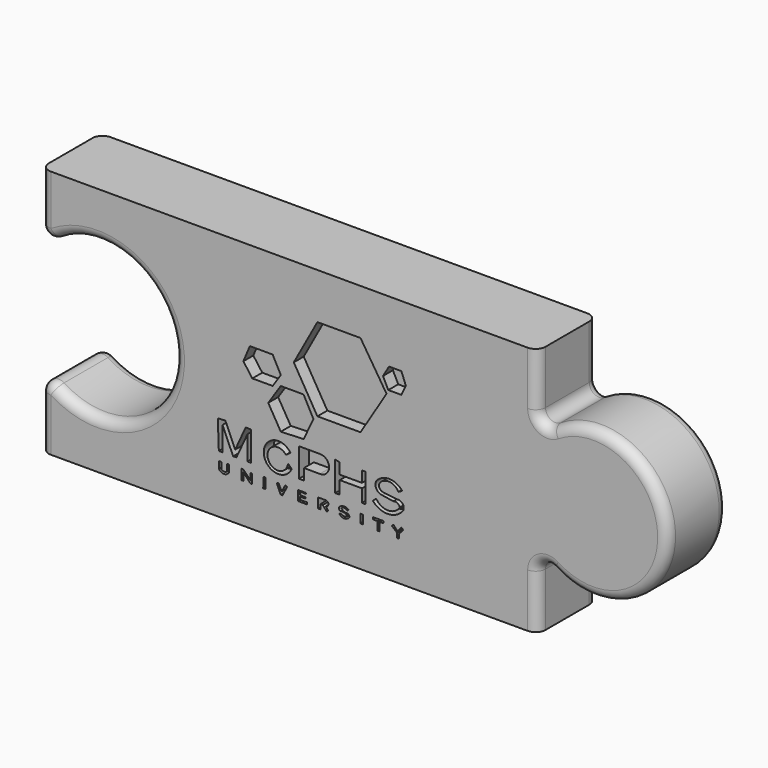
from build123d import *

# Parameters (mm, degrees)
F0_W     = 1.2396853417
F0_H     = 4.4274516404
F1_DEPTH = 38.1
F2_W     = 119.5903643966
F2_H     = 100.5869656801
F3_DEPTH = 31.75
F4_R     = 5.08
F5_F1_R  = 5.08
F5_F2_R  = 5.08


with BuildPart() as f1:
    # F0 (on Front) → F1 (new body)
    with BuildSketch(Plane.XZ):
        with BuildLine():
            Line((-152.3589964796, -18.4749997108), (-152.3589964796, -56.1939997108))
            Line((-152.3589964796, -56.1939997108), (101.6410035204, -56.1939997108))
            Line((101.6410035204, -56.1939997108), (101.6410035204, -17.8399997108))
            ThreePointArc((101.6410035204, -17.8399997108), (168.1390668347, 7.5600002892), (101.6410035204, 32.9600002892))
            Line((101.6410035204, 32.9600002892), (101.6410035204, 71.3140002892))
            Line((101.6410035204, 71.3140002892), (-152.3589964796, 71.3140002892))
            Line((-152.3589964796, 71.3140002892), (-152.3589964796, 34.8650002892))
            ThreePointArc((-152.3589964796, 34.8650002892), (-84.0285406821, 8.1950002892), (-152.3589964796, -18.4749997108))
        make_face()
        with BuildLine():
            Line((-61.3174373154, -34.5783394995), (-61.3174373154, -31.0568188551))
            Line((-61.3174373154, -31.0568188551), (-59.9337452893, -31.0568188551))
            Line((-59.9337452893, -31.0568188551), (-59.9337452893, -34.5783394995))
            ThreePointArc((-59.9337452893, -34.5783394995), (-58.6214708035, -34.9750876834), (-57.3091963177, -34.5783394995))
            Line((-57.3091963177, -34.5783394995), (-57.3091963177, -30.9339215281))
            Line((-57.3091963177, -30.9339215281), (-56.2031091993, -30.9339215281))
            Line((-56.2031091993, -30.9339215281), (-56.2031091993, -34.5783394995))
            ThreePointArc((-56.2031091993, -34.5783394995), (-58.7602732574, -36.0604791286), (-61.3174373154, -34.5783394995))
        make_face(mode=Mode.SUBTRACT)
        Polygon((-48.8504106049, -35.9585632804), (-49.8641850297, -35.9585632804), (-49.8641850297, -30.6131218794), (-48.8504106049, -30.7326440933), (-45.1566809659, -34.6184236231), (-45.1566809659, -31.1815415743), (-44.4813379888, -31.1815415743), (-44.4813379888, -35.9585632804), (-45.1566809659, -35.9585632804), (-48.8504106049, -32.0727837506), align=None, mode=Mode.SUBTRACT)
        Polygon((-37.5808859114, -35.9585632804), (-38.6635968332, -35.9585632804), (-38.5687844698, -30.7326440933), (-37.5808859114, -30.7326440933), align=None, mode=Mode.SUBTRACT)
        Polygon((-29.7552277202, -35.9585632804), (-31.7678497975, -31.3914579573), (-30.8955507223, -30.9392227448), (-29.1933210332, -34.3822178983), (-27.3931425903, -30.9392227448), (-26.4644501601, -31.4247918549), (-28.8349436466, -35.9585632804), align=None, mode=Mode.SUBTRACT)
        Polygon((-20.9552533795, -35.9585632804), (-20.9552533795, -30.9392227448), (-16.7476162185, -30.9392227448), (-16.7476162185, -31.4247918549), (-19.9163230006, -31.3914579573), (-19.9163230006, -32.909591985), (-16.9652923812, -32.909591985), (-16.9652923812, -33.6100806716), (-19.9163230006, -33.6100806716), (-19.9163230006, -35.0115646842), (-16.2226064001, -35.0115646842), (-16.2226064001, -35.9585632804), align=None, mode=Mode.SUBTRACT)
        with BuildLine():
            Line((-9.4527713825, -35.9585632804), (-10.54931454, -35.9585632804))
            Line((-10.54931454, -35.9585632804), (-10.54931454, -30.9392227448))
            Line((-10.54931454, -30.9392227448), (-6.6861817484, -30.9392227448))
            ThreePointArc((-6.6861817484, -30.9392227448), (-5.350752785, -32.2746517082), (-6.6861817484, -33.6100806716))
            Line((-6.6861817484, -33.6100806716), (-5.4284043645, -35.3105601402))
            Line((-5.4284043645, -35.3105601402), (-6.1631419683, -35.9585632804))
            Line((-6.1631419683, -35.9585632804), (-8.2343903939, -33.6100806716))
            Line((-8.2343903939, -33.6100806716), (-9.4527713825, -33.6100806716))
            Line((-9.4527713825, -33.6100806716), (-9.4527713825, -35.9585632804))
        make_face(mode=Mode.SUBTRACT)
        with BuildLine():
            ThreePointArc((4.3687420095, -35.5939765694), (2.0619009939, -36.0086349443), (0.2136342357, -34.5673275414))
            Line((0.2136342357, -34.5673275414), (1.3034986462, -34.5673275414))
            ThreePointArc((1.3034986462, -34.5673275414), (2.8361203279, -35.1923128719), (4.3687420095, -34.5673275414))
            ThreePointArc((4.3687420095, -34.5673275414), (2.9887125934, -33.5661164344), (1.3034986462, -33.3073524061))
            ThreePointArc((1.3034986462, -33.3073524061), (0.1017785642, -32.763786194), (0.4861005711, -31.502084178))
            ThreePointArc((0.4861005711, -31.502084178), (2.7680040932, -30.6538359895), (5.0499076153, -31.502084178))
            Line((5.0499076153, -31.502084178), (4.232510006, -32.0470159176))
            ThreePointArc((4.232510006, -32.0470159176), (2.7680043261, -31.2866876701), (1.3034986462, -32.0470159176))
            ThreePointArc((1.3034986462, -32.0470159176), (2.6880494547, -33.0373048641), (4.3687420095, -33.3073524061))
            ThreePointArc((4.3687420095, -33.3073524061), (5.3689469814, -34.4506644878), (4.3687420095, -35.5939765694))
        make_face(mode=Mode.SUBTRACT)
        Polygon((-59.4914490227, -26.5673523071), (-61.374177212, -26.5673523071), (-61.8983199651, -11.9427057781), (-58.0314019255, -11.8041166462), (-53.0015187031, -23.2180858651), (-47.6415390077, -11.5055379691), (-44.8480220382, -11.5055379691), (-44.8480220382, -26.5673523071), (-46.7307465021, -26.5673523071), (-46.7307465021, -14.225031552), (-52.3789273445, -26.5673523071), (-54.0524618571, -26.5673523071), (-59.4914490227, -14.225031552), align=None, mode=Mode.SUBTRACT)
        with BuildLine():
            ThreePointArc((-24.1380287205, -22.5927059772), (-38.3714144128, -20.264640143), (-24.7656023, -15.4801824364))
            Line((-24.7656023, -15.4801824364), (-27.0667122547, -17.1537188115))
            ThreePointArc((-27.0667122547, -17.1537188115), (-36.2738173156, -21.7936388182), (-26.0207531844, -20.7099796506))
            Line((-26.0207531844, -20.7099796506), (-24.1380287205, -22.5927059772))
        make_face(mode=Mode.SUBTRACT)
        with BuildLine():
            Line((-17.8622696419, -20.0775365629), (-17.8622696419, -25.7305850509))
            Line((-17.8622696419, -25.7305850509), (-20.3725714107, -25.7305850509))
            Line((-20.3725714107, -25.7305850509), (-20.3725714107, -11.087154341))
            Line((-20.3725714107, -11.087154341), (-9.4945952167, -11.087154341))
            ThreePointArc((-9.4945952167, -11.087154341), (-4.998187359, -15.6894044251), (-9.7037888934, -20.0775365629))
            Line((-9.7037888934, -20.0775365629), (-17.8622696419, -20.0775365629))
        make_face(mode=Mode.SUBTRACT)
        Polygon((0.3374228384, -11.4587976831), (0.3374228384, -17.1069794568), (11.8429763372, -17.1069794568), (11.8429763372, -11.4587976831), (13.5165052618, -11.4587976831), (13.5165052618, -26.148968679), (11.8429763372, -26.148968679), (11.8429763372, -19.5708436194), (0.4409505184, -19.5708436194), (0.4409505184, -26.148968679), (-1.8433485982, -26.148968679), (-1.8433485982, -11.1106832745), align=None, mode=Mode.SUBTRACT)
        Polygon((-18.0086121084, -7.1333109733), (-29.6823904039, -7.5516955327), (-36.1226030647, 3.3300416181), (-29.6823904039, 12.9903620513), (-18.0086121084, 12.9903620513), (-12.9880067082, 3.5354734067), align=None, mode=Mode.SUBTRACT)
        with Locations((11.6161257158, -33.429756132)):
            Rectangle(F0_W, F0_H, mode=Mode.SUBTRACT)
        Polygon((19.7745906319, -36.0482608202), (19.7745906319, -31.740860385), (17.5514137502, -31.740860385), (17.5514137502, -30.6987476769), (22.7619791533, -30.6987476769), (22.7619791533, -31.740860385), (20.8167014773, -31.740860385), (20.8167014773, -36.0482608202), align=None, mode=Mode.SUBTRACT)
        Polygon((29.7788707669, -33.7556128624), (27.0693777259, -31.4629649046), (27.9030678923, -30.6987476769), (29.9789267061, -32.9633172486), (31.94589076, -30.6987476769), (33.044158494, -31.4629649046), (30.7515105362, -33.8945624652), (30.7515105362, -36.1177374842), (29.7788707669, -36.1177374842), align=None, mode=Mode.SUBTRACT)
        with BuildLine():
            ThreePointArc((19.2863969262, -13.6697444367), (25.9430719524, -10.7785624658), (32.4211074169, -14.050459792))
            Line((32.4211074169, -14.050459792), (30.4447097978, -15.0999393715))
            ThreePointArc((30.4447097978, -15.0999393715), (26.0058375272, -12.0774565157), (21.0112156476, -14.050459792))
            ThreePointArc((21.0112156476, -14.050459792), (20.7189570122, -16.3618759907), (22.5675506647, -17.7798892001))
            Line((22.5675506647, -17.7798892001), (29.9174373253, -18.7042647275))
            ThreePointArc((29.9174373253, -18.7042647275), (32.8619726239, -20.1343754094), (32.4211074169, -23.3780064854))
            ThreePointArc((32.4211074169, -23.3780064854), (24.901962852, -26.814973044), (17.3828182872, -23.3780064854))
            Line((17.3828182872, -23.3780064854), (19.0960401799, -21.8551394763))
            ThreePointArc((19.0960401799, -21.8551394763), (25.1360740642, -25.2027143575), (31.1761079486, -21.8551394763))
            ThreePointArc((31.1761079486, -21.8551394763), (29.9174373253, -20.2960492657), (27.9170004781, -20.180869219))
            Line((27.9170004781, -20.180869219), (22.326243123, -19.3174825392))
            ThreePointArc((22.326243123, -19.3174825392), (19.1565421543, -17.3815921607), (19.2863969262, -13.6697444367))
        make_face(mode=Mode.SUBTRACT)
        Polygon((-48.817196873, 17.9166976962), (-45.4894024999, 25.8202028129), (-33.8421296449, 25.8202028129), (-29.6823904039, 17.9166976962), (-33.8421296449, 11.6770879034), (-44.241482404, 11.6770879034), align=None, mode=Mode.SUBTRACT)
        Polygon((-10.9635600941, 5.4374776449), (-23.0268072457, 25.8202028129), (-10.9635600941, 47.8668247018), (11.0830645888, 47.8668247018), (24.394230905, 27.0681247715), (11.0830645888, 5.4374776449), align=None, mode=Mode.SUBTRACT)
        Polygon((25.2941008537, 29.0568803105), (22.5746054082, 34.4958674762), (25.6562102466, 39.7593226884), (31.9882389037, 39.7593226884), (34.2893544464, 33.8682957593), (31.9882389037, 29.0568803105), align=None, mode=Mode.SUBTRACT)
    extrude(amount=F1_DEPTH)

    # F2 (on face) → F3 (join)
    with BuildSketch(Plane(origin=(0, 0, 0), x_dir=(-1, 0, 0), z_dir=(0, 1, 0))):
        with Locations((19.6628384292, 2.7849785984)):
            Rectangle(F2_W, F2_H)
    extrude(amount=-F3_DEPTH)

    # F4
    f4_edges = [f1.edges().sort_by_distance(p)[0] for p in [
        (-152.358996, -19.05, 34.865),
        (-84.028541, -38.1, 8.195),
        (-84.028541, 0, 8.195),
        (-152.358996, -19.05, -18.475),
        (-152.358996, -38.1, 53.0895),
        (-152.358996, -38.1, -37.3345),
        (-152.358996, 0, -37.3345),
        (-152.358996, 0, 53.0895),
    ]]
    fillet(f4_edges, radius=F4_R)

    # F5: fillet of radius 5.08 on 4 edges, made by hand

    # F5_f1
    f5_f1_edges = [f1.edges().sort_by_distance(p)[0] for p in [
        (101.6410035204, -19.05, 32.9600002892),
        (101.6410035204, -19.05, -17.8399997108),
    ]]
    fillet(f5_f1_edges, radius=F5_F1_R)

    # F5_f2
    f5_f2_edges = [f1.edges().sort_by_distance(p)[0] for p in [
        (168.1390668347, -38.1, 7.5600002892),
        (168.1390668347, 0, 7.5600002892),
        (104.2847740523, 0, -24.3248303738),
        (104.2847740523, 0, 39.4448309523),
        (104.2847740523, -38.1, -24.3248303738),
        (104.2847740523, -38.1, 39.4448309523),
    ]]
    fillet(f5_f2_edges, radius=F5_F2_R)


solid = f1.part
